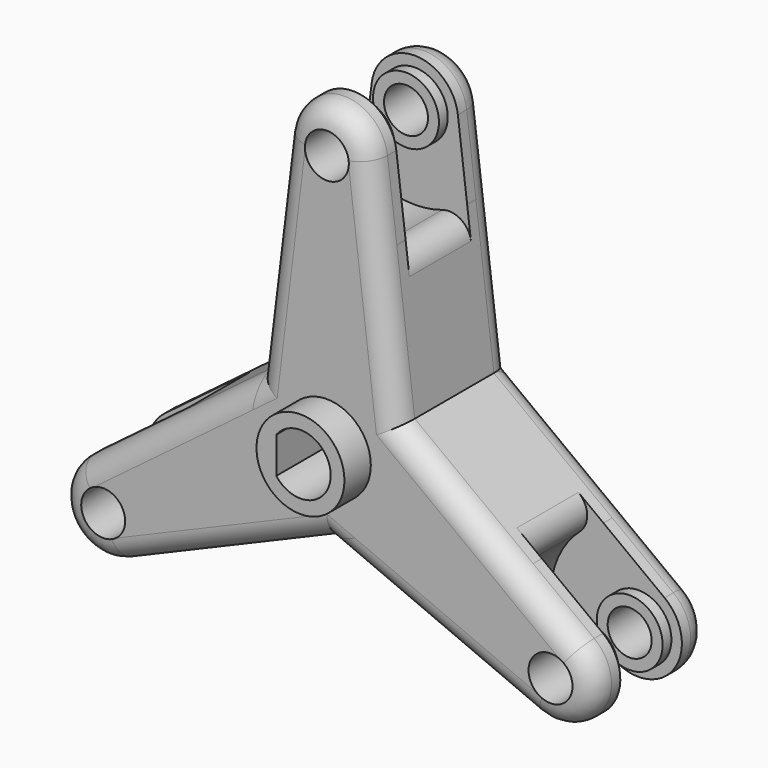
from build123d import *

# Parameters (mm, degrees)
F0_R          = 4
F0_R_2        = 3
F0_R_3        = 2
F1_DEPTH      = 13
F2_DEPTH      = 16
F3_START      = 3
F3_DEPTH      = 7
F4_START      = 4
F4_DEPTH      = 5
F5_T1_DEPTH   = 7
F5_T6_DEPTH   = 25.4355172255
F5_T11_DEPTH  = 25.4355172255
F5_T16_DEPTH  = 25.4355172255
F5_T21_DEPTH  = 25.4355172255
F5_T26_DEPTH  = 25.4355172255
F5_T31_DEPTH  = 25.4355172255
F5_T36_DEPTH  = 25.4355172255
F5_T39_ANGLE  = 166.0766048761
F5_T43_DEPTH  = 25.4355172255
F5_T46_ANGLE  = 166.0766048761
F5_T50_DEPTH  = 25.4355172255
F5_T53_ANGLE  = 166.0766048761
F5_T57_DEPTH  = 25.4355172255
F5_T62_DEPTH  = 25.4355172255
F5_T67_DEPTH  = 25.4355172255
F5_T70_ANGLE  = 166.0766048761
F5_T72_ANGLE  = 166.0766048761
F5_T74_ANGLE  = 166.0766048761
F5_T79_DEPTH  = 25.4355172255
F5_T83_DEPTH  = 25.4355172255
F5_T90_DEPTH  = 25.4355172255
F5_T94_DEPTH  = 25.4355172255
F5_T101_DEPTH = 25.4355172255
F5_T105_DEPTH = 25.4355172255
F5_T112_DEPTH = 25.4355172255
F5_T116_DEPTH = 25.4355172255
F5_T123_DEPTH = 25.4355172255
F5_T127_DEPTH = 25.4355172255
F5_T134_DEPTH = 25.4355172255
F5_T138_DEPTH = 25.4355172255


# Not quite as in the source:
# - a fillet or chamfer that OpenCascade refuses, or shapes differently, is made with other operations: its cross-section is extruded or revolved along the edge and cut away or added


with BuildPart() as f1:
    # F0 (on Front) → F1 (new body)
    with BuildSketch(Plane.XZ):
        Polygon((0, 8.5085643197), (-6.3981059606, 3.6939481987), (-7.3686328506, -4.2542821598), (0, -7.3878963973), (7.3686328506, -4.2542821598), (6.3981059606, 3.6939481987), align=None)
        Circle(F0_R, mode=Mode.SUBTRACT)
        with BuildLine():
            ThreePointArc((4.7643885892, 17.0734456066), (0, 15.5), (-4.7643885892, 17.0734456066))
            Line((-4.7643885892, 17.0734456066), (-6.3981059606, 3.6939481987))
            Line((-6.3981059606, 3.6939481987), (0, 8.5085643197))
            Line((0, 8.5085643197), (6.3981059606, 3.6939481987))
            Line((6.3981059606, 3.6939481987), (4.7643885892, 17.0734456066))
        make_face()
        with BuildLine():
            Line((17.1682319201, -4.4106412515), (6.3981059606, 3.6939481987))
            Line((6.3981059606, 3.6939481987), (7.3686328506, -4.2542821598))
            Line((7.3686328506, -4.2542821598), (0, -7.3878963973))
            Line((0, -7.3878963973), (12.4038433309, -12.6628043551))
            ThreePointArc((12.4038433309, -12.6628043551), (13.4233937587, -7.75), (17.1682319201, -4.4106412515))
        make_face()
        with BuildLine():
            Line((-7.3686328506, -4.2542821598), (-6.3981059606, 3.6939481987))
            Line((-6.3981059606, 3.6939481987), (-17.1682319201, -4.4106412515))
            ThreePointArc((-17.1682319201, -4.4106412515), (-13.4233937587, -7.75), (-12.4038433309, -12.6628043551))
            Line((-12.4038433309, -12.6628043551), (0, -7.3878963973))
            Line((0, -7.3878963973), (-7.3686328506, -4.2542821598))
        make_face()
        with BuildLine():
            Line((-3.921202839, 23.9788025289), (-4.7643885892, 17.0734456066))
            ThreePointArc((-4.7643885892, 17.0734456066), (0, 15.5), (4.7643885892, 17.0734456066))
            Line((4.7643885892, 17.0734456066), (3.921202839, 23.9788025289))
            ThreePointArc((3.921202839, 23.9788025289), (0, 27.4503270202), (-3.921202839, 23.9788025289))
        make_face()
        with Locations((0, 23.5)):
            Circle(F0_R_2, mode=Mode.SUBTRACT)
        with BuildLine():
            Line((22.7268535619, -8.5935399925), (17.1682319201, -4.4106412515))
            ThreePointArc((17.1682319201, -4.4106412515), (13.4233937587, -7.75), (12.4038433309, -12.6628043551))
            Line((12.4038433309, -12.6628043551), (18.8056507229, -15.3852625364))
            ThreePointArc((18.8056507229, -15.3852625364), (23.7726805417, -13.7251635101), (22.7268535619, -8.5935399925))
        make_face()
        with Locations((20.3515969889, -11.75)):
            Circle(F0_R_2, mode=Mode.SUBTRACT)
        with BuildLine():
            ThreePointArc((-12.4038433309, -12.6628043551), (-13.4233937587, -7.75), (-17.1682319201, -4.4106412515))
            Line((-17.1682319201, -4.4106412515), (-22.7268535619, -8.5935399925))
            ThreePointArc((-22.7268535619, -8.5935399925), (-23.7726805417, -13.7251635101), (-18.8056507229, -15.3852625364))
            Line((-18.8056507229, -15.3852625364), (-12.4038433309, -12.6628043551))
        make_face()
        with Locations((-20.3515969889, -11.75)):
            Circle(F0_R_2, mode=Mode.SUBTRACT)
        with Locations((0, 23.5)):
            Circle(F0_R_2)
        with Locations((0, 23.5)):
            Circle(F0_R_3, mode=Mode.SUBTRACT)
        with Locations((20.3515969889, -11.75)):
            Circle(F0_R_2)
        with Locations((20.3515969889, -11.75)):
            Circle(F0_R_3, mode=Mode.SUBTRACT)
        with Locations((-20.3515969889, -11.75)):
            Circle(F0_R_2)
        with Locations((-20.3515969889, -11.75)):
            Circle(F0_R_3, mode=Mode.SUBTRACT)
    extrude(amount=F1_DEPTH)

    # F0 (on Front) → F2 (join)
    with BuildSketch(Plane.XZ):
        Circle(F0_R)
        with BuildLine():
            ThreePointArc((-2.2, 1.65), (2.75, 0), (-2.2, -1.65))
            Line((-2.2, -1.65), (-2.2, 1.65))
        make_face(mode=Mode.SUBTRACT)
    extrude(amount=F2_DEPTH)

    # F0 (on Front) → F3 (cut)
    with BuildSketch(Plane.XZ.offset(F3_START)):
        with BuildLine():
            Line((-3.921202839, 23.9788025289), (-4.7643885892, 17.0734456066))
            ThreePointArc((-4.7643885892, 17.0734456066), (0, 15.5), (4.7643885892, 17.0734456066))
            Line((4.7643885892, 17.0734456066), (3.921202839, 23.9788025289))
            ThreePointArc((3.921202839, 23.9788025289), (0, 27.4503270202), (-3.921202839, 23.9788025289))
        make_face()
        with Locations((0, 23.5)):
            Circle(F0_R_2, mode=Mode.SUBTRACT)
        with BuildLine():
            ThreePointArc((-12.4038433309, -12.6628043551), (-13.4233937587, -7.75), (-17.1682319201, -4.4106412515))
            Line((-17.1682319201, -4.4106412515), (-22.7268535619, -8.5935399925))
            ThreePointArc((-22.7268535619, -8.5935399925), (-23.7726805417, -13.7251635101), (-18.8056507229, -15.3852625364))
            Line((-18.8056507229, -15.3852625364), (-12.4038433309, -12.6628043551))
        make_face()
        with Locations((-20.3515969889, -11.75)):
            Circle(F0_R_2, mode=Mode.SUBTRACT)
        with BuildLine():
            Line((22.7268535619, -8.5935399925), (17.1682319201, -4.4106412515))
            ThreePointArc((17.1682319201, -4.4106412515), (13.4233937587, -7.75), (12.4038433309, -12.6628043551))
            Line((12.4038433309, -12.6628043551), (18.8056507229, -15.3852625364))
            ThreePointArc((18.8056507229, -15.3852625364), (23.7726805417, -13.7251635101), (22.7268535619, -8.5935399925))
        make_face()
        with Locations((20.3515969889, -11.75)):
            Circle(F0_R_2, mode=Mode.SUBTRACT)
    extrude(amount=F3_DEPTH, mode=Mode.SUBTRACT)

    # F0 (on Front) → F4 (cut)
    with BuildSketch(Plane.XZ.offset(F4_START)):
        with Locations((0, 23.5)):
            Circle(F0_R_2)
        with Locations((0, 23.5)):
            Circle(F0_R_3, mode=Mode.SUBTRACT)
        with Locations((-20.3515969889, -11.75)):
            Circle(F0_R_2)
        with Locations((-20.3515969889, -11.75)):
            Circle(F0_R_3, mode=Mode.SUBTRACT)
        with Locations((20.3515969889, -11.75)):
            Circle(F0_R_2)
        with Locations((20.3515969889, -11.75)):
            Circle(F0_R_3, mode=Mode.SUBTRACT)
    extrude(amount=F4_DEPTH, mode=Mode.SUBTRACT)

    # F5: fillet of radius 2 on 24 edges, made by hand

    # F5_s2 → F5_t1 (cut)
    with BuildSketch(Plane.XZ.offset(3)):
        with BuildLine():
            ThreePointArc((5.1099853299, 14.2431453501), (4.1968257437, 15.6891092661), (2.499784424, 15.9005870073))
            ThreePointArc((2.499784424, 15.9005870073), (3.67912377, 16.3961948024), (4.7643885892, 17.0734456066))
            Line((4.7643885892, 17.0734456066), (5.1099853299, 14.2431453501))
        make_face()
        with BuildLine():
            ThreePointArc((14.8899183679, -2.6961955664), (15.6855800591, -4.2099969237), (15.0202044954, -5.7854166885))
            ThreePointArc((15.0202044954, -5.7854166885), (16.0390831093, -5.0118827527), (17.1682319201, -4.4106412515))
            Line((17.1682319201, -4.4106412515), (14.8899183679, -2.6961955664))
        make_face()
        with BuildLine():
            ThreePointArc((-9.7799330381, -11.5469497837), (-11.4887543153, -11.4791123424), (-12.5204200714, -10.1151703188))
            ThreePointArc((-12.5204200714, -10.1151703188), (-12.3599593393, -11.3843120497), (-12.4038433309, -12.6628043551))
            Line((-12.4038433309, -12.6628043551), (-9.7799330381, -11.5469497837))
        make_face()
        with BuildLine():
            ThreePointArc((-14.8899183679, -2.6961955664), (-15.6855800591, -4.2099969237), (-15.0202044954, -5.7854166885))
            ThreePointArc((-15.0202044954, -5.7854166885), (-16.0390831093, -5.0118827527), (-17.1682319201, -4.4106412515))
            Line((-17.1682319201, -4.4106412515), (-14.8899183679, -2.6961955664))
        make_face()
        with BuildLine():
            ThreePointArc((-5.1099853299, 14.2431453501), (-4.1968257437, 15.6891092661), (-2.499784424, 15.9005870073))
            ThreePointArc((-2.499784424, 15.9005870073), (-3.67912377, 16.3961948024), (-4.7643885892, 17.0734456066))
            Line((-4.7643885892, 17.0734456066), (-5.1099853299, 14.2431453501))
        make_face()
        with BuildLine():
            ThreePointArc((9.7799330381, -11.5469497837), (11.4887543153, -11.4791123424), (12.5204200714, -10.1151703188))
            ThreePointArc((12.5204200714, -10.1151703188), (12.3599593393, -11.3843120497), (12.4038433309, -12.6628043551))
            Line((12.4038433309, -12.6628043551), (9.7799330381, -11.5469497837))
        make_face()
    extrude(amount=F5_T1_DEPTH, mode=Mode.SUBTRACT)


with BuildPart() as f5_tool4:
    # F5_s5 → F5_t6 (new body)
    with BuildSketch(Plane(origin=(2.8273365505, 0, 23.1547651458), x_dir=(0, 1, 0), z_dir=(-0.1212057955, 0, -0.9926274))):
        with BuildLine():
            ThreePointArc((-11, -6.7986632142), (-12.4142135624, -6.2128767766), (-13, -4.7986632142))
            Line((-13, -4.7986632142), (-13, -6.7986632142))
            Line((-13, -6.7986632142), (-11, -6.7986632142))
        make_face()
    extrude(amount=F5_T6_DEPTH)

    split(bisect_by=Plane(origin=(-4.0879070023, 0, 5.4323878582), x_dir=(0, 1, 0), z_dir=(-0.601280998, 0, 0.7990376471)), keep=Keep.TOP)


with BuildPart() as f1_1:
    add(f1.part)

    # F5_t3: cut F5_tool4
    add(f5_tool4.part, mode=Mode.SUBTRACT)


with BuildPart() as f5_tool9:
    # F5_s10 → F5_t11 (new body)
    with BuildSketch(Plane(origin=(18.6389465596, 0, -14.0259278507), x_dir=(0, 1, 0), z_dir=(-0.7990376471, 0, 0.601280998))):
        with BuildLine():
            ThreePointArc((-11, -6.7986632142), (-12.4142135624, -6.2128767766), (-13, -4.7986632142))
            Line((-13, -4.7986632142), (-13, -6.7986632142))
            Line((-13, -6.7986632142), (-11, -6.7986632142))
        make_face()
    extrude(amount=F5_T11_DEPTH)

    split(bisect_by=Plane(origin=(6.7485393895, 0, 0.8240373832), x_dir=(0, 1, 0), z_dir=(0.9926274, 0, 0.1212057955)), keep=Keep.TOP)


with BuildPart() as f1_2:
    add(f1_1.part)

    # F5_t8: cut F5_tool9
    add(f5_tool9.part, mode=Mode.SUBTRACT)


with BuildPart() as f5_tool14:
    # F5_s15 → F5_t16 (new body)
    with BuildSketch(Plane(origin=(-21.4662831102, 0, -9.1288372951), x_dir=(0, 1, 0), z_dir=(0.9202434426, 0, 0.391346402))):
        with BuildLine():
            ThreePointArc((-11, -6.7986632142), (-12.4142135624, -6.2128767766), (-13, -4.7986632142))
            Line((-13, -4.7986632142), (-13, -6.7986632142))
            Line((-13, -6.7986632142), (-11, -6.7986632142))
        make_face()
    extrude(amount=F5_T16_DEPTH)

    split(bisect_by=Plane(origin=(-2.6606323873, 0, -6.2564252413), x_dir=(0, 1, 0), z_dir=(-0.391346402, 0, -0.9202434426)), keep=Keep.TOP)


with BuildPart() as f1_3:
    add(f1_2.part)

    # F5_t13: cut F5_tool14
    add(f5_tool14.part, mode=Mode.SUBTRACT)


with BuildPart() as f5_tool19:
    # F5_s20 → F5_t21 (new body)
    with BuildSketch(Plane(origin=(0.2555955486, 0, -2.0932261843), x_dir=(0, 1, 0), z_dir=(-0.1212057955, 0, 0.9926274))):
        with BuildLine():
            ThreePointArc((0, -4.7986632142), (-0.5857864376, -6.2128767766), (-2, -6.7986632142))
            Line((-2, -6.7986632142), (0, -6.7986632142))
            Line((0, -6.7986632142), (0, -4.7986632142))
        make_face()
    extrude(amount=F5_T21_DEPTH)

    split(bisect_by=Plane(origin=(4.0879070023, 0, 5.4323878582), x_dir=(0, 1, 0), z_dir=(0.601280998, 0, 0.7990376471)), keep=Keep.TOP)


with BuildPart() as f1_4:
    add(f1_3.part)

    # F5_t18: cut F5_tool19
    add(f5_tool19.part, mode=Mode.SUBTRACT)


with BuildPart() as f5_tool24:
    # F5_s25 → F5_t26 (new body)
    with BuildSketch(Plane(origin=(1.6849892772, 0, 1.2679653303), x_dir=(0, 1, 0), z_dir=(-0.7990376471, 0, -0.601280998))):
        with BuildLine():
            ThreePointArc((0, -4.7986632142), (-0.5857864376, -6.2128767766), (-2, -6.7986632142))
            Line((-2, -6.7986632142), (0, -6.7986632142))
            Line((0, -6.7986632142), (0, -4.7986632142))
        make_face()
    extrude(amount=F5_T26_DEPTH)

    split(bisect_by=Plane(origin=(-6.7485393895, 0, 0.8240373832), x_dir=(0, 1, 0), z_dir=(-0.9926274, 0, 0.1212057955)), keep=Keep.TOP)


with BuildPart() as f1_5:
    add(f1_4.part)

    # F5_t23: cut F5_tool24
    add(f5_tool24.part, mode=Mode.SUBTRACT)


with BuildPart() as f5_tool29:
    # F5_s30 → F5_t31 (new body)
    with BuildSketch(Plane(origin=(-1.9405848257, 0, 0.825260854), x_dir=(0, 1, 0), z_dir=(0.9202434426, 0, -0.391346402))):
        with BuildLine():
            ThreePointArc((0, -4.7986632142), (-0.5857864376, -6.2128767766), (-2, -6.7986632142))
            Line((-2, -6.7986632142), (0, -6.7986632142))
            Line((0, -6.7986632142), (0, -4.7986632142))
        make_face()
    extrude(amount=F5_T31_DEPTH)

    split(bisect_by=Plane(origin=(2.6606323873, 0, -6.2564252413), x_dir=(0, 1, 0), z_dir=(0.391346402, 0, -0.9202434426)), keep=Keep.TOP)


with BuildPart() as f1_6:
    add(f1_5.part)

    # F5_t28: cut F5_tool29
    add(f5_tool29.part, mode=Mode.SUBTRACT)


with BuildPart() as f5_tool34:
    # F5_s35 → F5_t36 (new body)
    with BuildSketch(Plane(origin=(2.8273365505, 0, 23.1547651458), x_dir=(0, 1, 0), z_dir=(-0.1212057955, 0, -0.9926274))):
        with BuildLine():
            ThreePointArc((0, -4.7986632142), (-0.5857864376, -6.2128767766), (-2, -6.7986632142))
            Line((-2, -6.7986632142), (0, -6.7986632142))
            Line((0, -6.7986632142), (0, -4.7986632142))
        make_face()
    extrude(amount=F5_T36_DEPTH)

    split(bisect_by=Plane(origin=(-4.0879070023, 0, 5.4323878582), x_dir=(0, 1, 0), z_dir=(-0.601280998, 0, 0.7990376471)), keep=Keep.TOP)


with BuildPart() as f1_7:
    add(f1_6.part)

    # F5_t33: cut F5_tool34
    add(f5_tool34.part, mode=Mode.SUBTRACT)

    # F5_s38 → F5_t39 (revolve, cut)
    with BuildSketch(Plane(origin=(-18.6389465596, 0, -14.0259278507), x_dir=(0, 1, 0), z_dir=(0.7990376471, 0, 0.601280998))):
        with BuildLine():
            ThreePointArc((0, 4.7986632142), (-0.5857864376, 6.2128767766), (-2, 6.7986632142))
            Line((-2, 6.7986632142), (0, 6.7986632142))
            Line((0, 6.7986632142), (0, 4.7986632142))
        make_face()
    revolve(axis=Axis((-20.3515969889, 0, -11.75), (0, -1, 0)), revolution_arc=F5_T39_ANGLE, mode=Mode.SUBTRACT)


with BuildPart() as f5_tool41:
    # F5_s42 → F5_t43 (new body)
    with BuildSketch(Plane(origin=(-21.4662831102, 0, -9.1288372951), x_dir=(0, 1, 0), z_dir=(0.9202434426, 0, 0.391346402))):
        with BuildLine():
            ThreePointArc((0, -4.7986632142), (-0.5857864376, -6.2128767766), (-2, -6.7986632142))
            Line((-2, -6.7986632142), (0, -6.7986632142))
            Line((0, -6.7986632142), (0, -4.7986632142))
        make_face()
    extrude(amount=F5_T43_DEPTH)

    split(bisect_by=Plane(origin=(-2.6606323873, 0, -6.2564252413), x_dir=(0, 1, 0), z_dir=(-0.391346402, 0, -0.9202434426)), keep=Keep.TOP)


with BuildPart() as f1_8:
    add(f1_7.part)

    # F5_t40: cut F5_tool41
    add(f5_tool41.part, mode=Mode.SUBTRACT)

    # F5_s45 → F5_t46 (revolve, cut)
    with BuildSketch(Plane(origin=(21.4662831102, 0, -9.1288372951), x_dir=(0, 1, 0), z_dir=(-0.9202434426, 0, 0.391346402))):
        with BuildLine():
            ThreePointArc((0, 4.7986632142), (-0.5857864376, 6.2128767766), (-2, 6.7986632142))
            Line((-2, 6.7986632142), (0, 6.7986632142))
            Line((0, 6.7986632142), (0, 4.7986632142))
        make_face()
    revolve(axis=Axis((20.3515969889, 0, -11.75), (0, -1, 0)), revolution_arc=F5_T46_ANGLE, mode=Mode.SUBTRACT)


with BuildPart() as f5_tool48:
    # F5_s49 → F5_t50 (new body)
    with BuildSketch(Plane(origin=(18.6389465596, 0, -14.0259278507), x_dir=(0, 1, 0), z_dir=(-0.7990376471, 0, 0.601280998))):
        with BuildLine():
            ThreePointArc((0, -4.7986632142), (-0.5857864376, -6.2128767766), (-2, -6.7986632142))
            Line((-2, -6.7986632142), (0, -6.7986632142))
            Line((0, -6.7986632142), (0, -4.7986632142))
        make_face()
    extrude(amount=F5_T50_DEPTH)

    split(bisect_by=Plane(origin=(6.7485393895, 0, 0.8240373832), x_dir=(0, 1, 0), z_dir=(0.9926274, 0, 0.1212057955)), keep=Keep.TOP)


with BuildPart() as f1_9:
    add(f1_8.part)

    # F5_t47: cut F5_tool48
    add(f5_tool48.part, mode=Mode.SUBTRACT)

    # F5_s52 → F5_t53 (revolve, cut)
    with BuildSketch(Plane(origin=(-2.8273365505, 0, 23.1547651458), x_dir=(0, 1, 0), z_dir=(0.1212057955, 0, -0.9926274))):
        with BuildLine():
            ThreePointArc((0, 4.7986632142), (-0.5857864376, 6.2128767766), (-2, 6.7986632142))
            Line((-2, 6.7986632142), (0, 6.7986632142))
            Line((0, 6.7986632142), (0, 4.7986632142))
        make_face()
    revolve(axis=Axis((0, 0, 23.5), (0, -1, 0)), revolution_arc=F5_T53_ANGLE, mode=Mode.SUBTRACT)


with BuildPart() as f5_tool55:
    # F5_s56 → F5_t57 (new body)
    with BuildSketch(Plane(origin=(1.6849892772, 0, 1.2679653303), x_dir=(0, 1, 0), z_dir=(-0.7990376471, 0, -0.601280998))):
        with BuildLine():
            ThreePointArc((-11, -6.7986632142), (-12.4142135624, -6.2128767766), (-13, -4.7986632142))
            Line((-13, -4.7986632142), (-13, -6.7986632142))
            Line((-13, -6.7986632142), (-11, -6.7986632142))
        make_face()
    extrude(amount=F5_T57_DEPTH)

    split(bisect_by=Plane(origin=(-6.7485393895, 0, 0.8240373832), x_dir=(0, 1, 0), z_dir=(-0.9926274, 0, 0.1212057955)), keep=Keep.TOP)


with BuildPart() as f1_10:
    add(f1_9.part)

    # F5_t54: cut F5_tool55
    add(f5_tool55.part, mode=Mode.SUBTRACT)


with BuildPart() as f5_tool60:
    # F5_s61 → F5_t62 (new body)
    with BuildSketch(Plane(origin=(-1.9405848257, 0, 0.825260854), x_dir=(0, 1, 0), z_dir=(0.9202434426, 0, -0.391346402))):
        with BuildLine():
            ThreePointArc((-11, -6.7986632142), (-12.4142135624, -6.2128767766), (-13, -4.7986632142))
            Line((-13, -4.7986632142), (-13, -6.7986632142))
            Line((-13, -6.7986632142), (-11, -6.7986632142))
        make_face()
    extrude(amount=F5_T62_DEPTH)

    split(bisect_by=Plane(origin=(2.6606323873, 0, -6.2564252413), x_dir=(0, 1, 0), z_dir=(0.391346402, 0, -0.9202434426)), keep=Keep.TOP)


with BuildPart() as f1_11:
    add(f1_10.part)

    # F5_t59: cut F5_tool60
    add(f5_tool60.part, mode=Mode.SUBTRACT)


with BuildPart() as f5_tool65:
    # F5_s66 → F5_t67 (new body)
    with BuildSketch(Plane(origin=(0.2555955486, 0, -2.0932261843), x_dir=(0, 1, 0), z_dir=(-0.1212057955, 0, 0.9926274))):
        with BuildLine():
            ThreePointArc((-11, -6.7986632142), (-12.4142135624, -6.2128767766), (-13, -4.7986632142))
            Line((-13, -4.7986632142), (-13, -6.7986632142))
            Line((-13, -6.7986632142), (-11, -6.7986632142))
        make_face()
    extrude(amount=F5_T67_DEPTH)

    split(bisect_by=Plane(origin=(4.0879070023, 0, 5.4323878582), x_dir=(0, 1, 0), z_dir=(0.601280998, 0, 0.7990376471)), keep=Keep.TOP)


with BuildPart() as f1_12:
    add(f1_11.part)

    # F5_t64: cut F5_tool65
    add(f5_tool65.part, mode=Mode.SUBTRACT)

    # F5_s69 → F5_t70 (revolve, cut)
    with BuildSketch(Plane(origin=(-18.6389465596, 0, -14.0259278507), x_dir=(0, 1, 0), z_dir=(0.7990376471, 0, 0.601280998))):
        with BuildLine():
            ThreePointArc((-13, 4.7986632142), (-12.4142135624, 6.2128767766), (-11, 6.7986632142))
            Line((-11, 6.7986632142), (-13, 6.7986632142))
            Line((-13, 6.7986632142), (-13, 4.7986632142))
        make_face()
    revolve(axis=Axis((-20.3515969889, -13, -11.75), (0, -1, 0)), revolution_arc=F5_T70_ANGLE, mode=Mode.SUBTRACT)

    # F5_s71 → F5_t72 (revolve, cut)
    with BuildSketch(Plane(origin=(21.4662831102, 0, -9.1288372951), x_dir=(0, 1, 0), z_dir=(-0.9202434426, 0, 0.391346402))):
        with BuildLine():
            ThreePointArc((-13, 4.7986632142), (-12.4142135624, 6.2128767766), (-11, 6.7986632142))
            Line((-11, 6.7986632142), (-13, 6.7986632142))
            Line((-13, 6.7986632142), (-13, 4.7986632142))
        make_face()
    revolve(axis=Axis((20.3515969889, -13, -11.75), (0, -1, 0)), revolution_arc=F5_T72_ANGLE, mode=Mode.SUBTRACT)

    # F5_s73 → F5_t74 (revolve, cut)
    with BuildSketch(Plane(origin=(-2.8273365505, 0, 23.1547651458), x_dir=(0, 1, 0), z_dir=(0.1212057955, 0, -0.9926274))):
        with BuildLine():
            ThreePointArc((-13, 4.7986632142), (-12.4142135624, 6.2128767766), (-11, 6.7986632142))
            Line((-11, 6.7986632142), (-13, 6.7986632142))
            Line((-13, 6.7986632142), (-13, 4.7986632142))
        make_face()
    revolve(axis=Axis((0, -13, 23.5), (0, -1, 0)), revolution_arc=F5_T74_ANGLE, mode=Mode.SUBTRACT)


with BuildPart() as f5_tool77:
    # F5_s78 → F5_t79 (new body)
    with BuildSketch(Plane(origin=(2.8273365505, 0, 23.1547651458), x_dir=(0, 1, 0), z_dir=(-0.1212057955, 0, -0.9926274))):
        with BuildLine():
            ThreePointArc((-11, -6.7986632142), (-12.4142135624, -6.2128767766), (-13, -4.7986632142))
            Line((-13, -4.7986632142), (-13, -6.7986632142))
            Line((-13, -6.7986632142), (-11, -6.7986632142))
        make_face()
    extrude(amount=F5_T79_DEPTH)

    split(bisect_by=Plane(origin=(-4.0879070023, 0, 5.4323878582), x_dir=(0, 1, 0), z_dir=(0.601280998, 0, -0.7990376471)), keep=Keep.TOP)


with BuildPart() as f5_tool81:
    # F5_s82 → F5_t83 (new body)
    with BuildSketch(Plane(origin=(1.6849892772, 0, 1.2679653303), x_dir=(0, 1, 0), z_dir=(-0.7990376471, 0, -0.601280998))):
        with BuildLine():
            ThreePointArc((-11, -6.7986632142), (-12.4142135624, -6.2128767766), (-13, -4.7986632142))
            Line((-13, -4.7986632142), (-13, -6.7986632142))
            Line((-13, -6.7986632142), (-11, -6.7986632142))
        make_face()
    extrude(amount=F5_T83_DEPTH)

    split(bisect_by=Plane(origin=(-6.7485393895, 0, 0.8240373832), x_dir=(0, 1, 0), z_dir=(0.9926274, 0, -0.1212057955)), keep=Keep.TOP)


with BuildPart() as f5_tool77_1:
    add(f5_tool77.part)

    # F5_t85: intersect F5_tool81
    add(f5_tool81.part, mode=Mode.INTERSECT)


with BuildPart() as f1_13:
    add(f1_12.part)

    # F5_t75: cut F5_tool77
    add(f5_tool77_1.part, mode=Mode.SUBTRACT)


with BuildPart() as f5_tool88:
    # F5_s89 → F5_t90 (new body)
    with BuildSketch(Plane(origin=(18.6389465596, 0, -14.0259278507), x_dir=(0, 1, 0), z_dir=(-0.7990376471, 0, 0.601280998))):
        with BuildLine():
            ThreePointArc((-11, -6.7986632142), (-12.4142135624, -6.2128767766), (-13, -4.7986632142))
            Line((-13, -4.7986632142), (-13, -6.7986632142))
            Line((-13, -6.7986632142), (-11, -6.7986632142))
        make_face()
    extrude(amount=F5_T90_DEPTH)

    split(bisect_by=Plane(origin=(6.7485393895, 0, 0.8240373832), x_dir=(0, 1, 0), z_dir=(-0.9926274, 0, -0.1212057955)), keep=Keep.TOP)


with BuildPart() as f5_tool92:
    # F5_s93 → F5_t94 (new body)
    with BuildSketch(Plane(origin=(0.2555955486, 0, -2.0932261843), x_dir=(0, 1, 0), z_dir=(-0.1212057955, 0, 0.9926274))):
        with BuildLine():
            ThreePointArc((-11, -6.7986632142), (-12.4142135624, -6.2128767766), (-13, -4.7986632142))
            Line((-13, -4.7986632142), (-13, -6.7986632142))
            Line((-13, -6.7986632142), (-11, -6.7986632142))
        make_face()
    extrude(amount=F5_T94_DEPTH)

    split(bisect_by=Plane(origin=(4.0879070023, 0, 5.4323878582), x_dir=(0, 1, 0), z_dir=(-0.601280998, 0, -0.7990376471)), keep=Keep.TOP)


with BuildPart() as f5_tool88_1:
    add(f5_tool88.part)

    # F5_t96: intersect F5_tool92
    add(f5_tool92.part, mode=Mode.INTERSECT)


with BuildPart() as f1_14:
    add(f1_13.part)

    # F5_t86: cut F5_tool88
    add(f5_tool88_1.part, mode=Mode.SUBTRACT)


with BuildPart() as f5_tool99:
    # F5_s100 → F5_t101 (new body)
    with BuildSketch(Plane(origin=(-21.4662831102, 0, -9.1288372951), x_dir=(0, 1, 0), z_dir=(0.9202434426, 0, 0.391346402))):
        with BuildLine():
            ThreePointArc((-11, -6.7986632142), (-12.4142135624, -6.2128767766), (-13, -4.7986632142))
            Line((-13, -4.7986632142), (-13, -6.7986632142))
            Line((-13, -6.7986632142), (-11, -6.7986632142))
        make_face()
    extrude(amount=F5_T101_DEPTH)

    split(bisect_by=Plane(origin=(-2.6606323873, 0, -6.2564252413), x_dir=(0, 1, 0), z_dir=(0.391346402, 0, 0.9202434426)), keep=Keep.TOP)


with BuildPart() as f5_tool103:
    # F5_s104 → F5_t105 (new body)
    with BuildSketch(Plane(origin=(-1.9405848257, 0, 0.825260854), x_dir=(0, 1, 0), z_dir=(0.9202434426, 0, -0.391346402))):
        with BuildLine():
            ThreePointArc((-11, -6.7986632142), (-12.4142135624, -6.2128767766), (-13, -4.7986632142))
            Line((-13, -4.7986632142), (-13, -6.7986632142))
            Line((-13, -6.7986632142), (-11, -6.7986632142))
        make_face()
    extrude(amount=F5_T105_DEPTH)

    split(bisect_by=Plane(origin=(2.6606323873, 0, -6.2564252413), x_dir=(0, 1, 0), z_dir=(-0.391346402, 0, 0.9202434426)), keep=Keep.TOP)


with BuildPart() as f5_tool99_1:
    add(f5_tool99.part)

    # F5_t107: intersect F5_tool103
    add(f5_tool103.part, mode=Mode.INTERSECT)


with BuildPart() as f1_15:
    add(f1_14.part)

    # F5_t97: cut F5_tool99
    add(f5_tool99_1.part, mode=Mode.SUBTRACT)


with BuildPart() as f5_tool110:
    # F5_s111 → F5_t112 (new body)
    with BuildSketch(Plane(origin=(18.6389465596, 0, -14.0259278507), x_dir=(0, 1, 0), z_dir=(-0.7990376471, 0, 0.601280998))):
        with BuildLine():
            ThreePointArc((0, -4.7986632142), (-0.5857864376, -6.2128767766), (-2, -6.7986632142))
            Line((-2, -6.7986632142), (0, -6.7986632142))
            Line((0, -6.7986632142), (0, -4.7986632142))
        make_face()
    extrude(amount=F5_T112_DEPTH)

    split(bisect_by=Plane(origin=(6.7485393895, 0, 0.8240373832), x_dir=(0, 1, 0), z_dir=(-0.9926274, 0, -0.1212057955)), keep=Keep.TOP)


with BuildPart() as f5_tool114:
    # F5_s115 → F5_t116 (new body)
    with BuildSketch(Plane(origin=(0.2555955486, 0, -2.0932261843), x_dir=(0, 1, 0), z_dir=(-0.1212057955, 0, 0.9926274))):
        with BuildLine():
            ThreePointArc((0, -4.7986632142), (-0.5857864376, -6.2128767766), (-2, -6.7986632142))
            Line((-2, -6.7986632142), (0, -6.7986632142))
            Line((0, -6.7986632142), (0, -4.7986632142))
        make_face()
    extrude(amount=F5_T116_DEPTH)

    split(bisect_by=Plane(origin=(4.0879070023, 0, 5.4323878582), x_dir=(0, 1, 0), z_dir=(-0.601280998, 0, -0.7990376471)), keep=Keep.TOP)


with BuildPart() as f5_tool110_1:
    add(f5_tool110.part)

    # F5_t118: intersect F5_tool114
    add(f5_tool114.part, mode=Mode.INTERSECT)


with BuildPart() as f1_16:
    add(f1_15.part)

    # F5_t108: cut F5_tool110
    add(f5_tool110_1.part, mode=Mode.SUBTRACT)


with BuildPart() as f5_tool121:
    # F5_s122 → F5_t123 (new body)
    with BuildSketch(Plane(origin=(2.8273365505, 0, 23.1547651458), x_dir=(0, 1, 0), z_dir=(-0.1212057955, 0, -0.9926274))):
        with BuildLine():
            ThreePointArc((0, -4.7986632142), (-0.5857864376, -6.2128767766), (-2, -6.7986632142))
            Line((-2, -6.7986632142), (0, -6.7986632142))
            Line((0, -6.7986632142), (0, -4.7986632142))
        make_face()
    extrude(amount=F5_T123_DEPTH)

    split(bisect_by=Plane(origin=(-4.0879070023, 0, 5.4323878582), x_dir=(0, 1, 0), z_dir=(0.601280998, 0, -0.7990376471)), keep=Keep.TOP)


with BuildPart() as f5_tool125:
    # F5_s126 → F5_t127 (new body)
    with BuildSketch(Plane(origin=(1.6849892772, 0, 1.2679653303), x_dir=(0, 1, 0), z_dir=(-0.7990376471, 0, -0.601280998))):
        with BuildLine():
            ThreePointArc((0, -4.7986632142), (-0.5857864376, -6.2128767766), (-2, -6.7986632142))
            Line((-2, -6.7986632142), (0, -6.7986632142))
            Line((0, -6.7986632142), (0, -4.7986632142))
        make_face()
    extrude(amount=F5_T127_DEPTH)

    split(bisect_by=Plane(origin=(-6.7485393895, 0, 0.8240373832), x_dir=(0, 1, 0), z_dir=(0.9926274, 0, -0.1212057955)), keep=Keep.TOP)


with BuildPart() as f5_tool121_1:
    add(f5_tool121.part)

    # F5_t129: intersect F5_tool125
    add(f5_tool125.part, mode=Mode.INTERSECT)


with BuildPart() as f1_17:
    add(f1_16.part)

    # F5_t119: cut F5_tool121
    add(f5_tool121_1.part, mode=Mode.SUBTRACT)


with BuildPart() as f5_tool132:
    # F5_s133 → F5_t134 (new body)
    with BuildSketch(Plane(origin=(-21.4662831102, 0, -9.1288372951), x_dir=(0, 1, 0), z_dir=(0.9202434426, 0, 0.391346402))):
        with BuildLine():
            ThreePointArc((0, -4.7986632142), (-0.5857864376, -6.2128767766), (-2, -6.7986632142))
            Line((-2, -6.7986632142), (0, -6.7986632142))
            Line((0, -6.7986632142), (0, -4.7986632142))
        make_face()
    extrude(amount=F5_T134_DEPTH)

    split(bisect_by=Plane(origin=(-2.6606323873, 0, -6.2564252413), x_dir=(0, 1, 0), z_dir=(0.391346402, 0, 0.9202434426)), keep=Keep.TOP)


with BuildPart() as f5_tool136:
    # F5_s137 → F5_t138 (new body)
    with BuildSketch(Plane(origin=(-1.9405848257, 0, 0.825260854), x_dir=(0, 1, 0), z_dir=(0.9202434426, 0, -0.391346402))):
        with BuildLine():
            ThreePointArc((0, -4.7986632142), (-0.5857864376, -6.2128767766), (-2, -6.7986632142))
            Line((-2, -6.7986632142), (0, -6.7986632142))
            Line((0, -6.7986632142), (0, -4.7986632142))
        make_face()
    extrude(amount=F5_T138_DEPTH)

    split(bisect_by=Plane(origin=(2.6606323873, 0, -6.2564252413), x_dir=(0, 1, 0), z_dir=(-0.391346402, 0, 0.9202434426)), keep=Keep.TOP)


with BuildPart() as f5_tool132_1:
    add(f5_tool132.part)

    # F5_t140: intersect F5_tool136
    add(f5_tool136.part, mode=Mode.INTERSECT)


with BuildPart() as f1_18:
    add(f1_17.part)

    # F5_t130: cut F5_tool132
    add(f5_tool132_1.part, mode=Mode.SUBTRACT)


solid = f1_18.part
